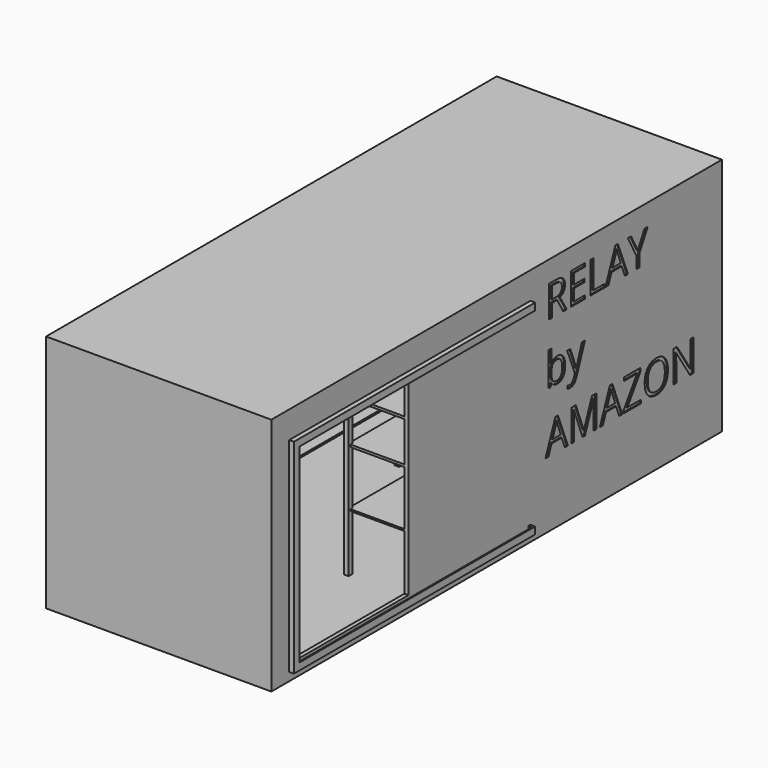
from build123d import *

# Parameters (mm, degrees)
F0_W          = 2438.4
F0_H          = 2590.8
F0_W_2        = 2352.04
F0_H_2        = 2395.22
F1_DEPTH      = 6096
F2_W          = 2352.04
F2_H          = 2395.22
F3_DEPTH      = 127
F4_W          = 2352.04
F4_H          = 2395.22
F5_DEPTH      = 127
F6_W          = 1524
F6_H          = 2032
F7_DEPTH      = 50.8
F9_DEPTH      = 50.8
F11_DEPTH     = 38.1
F12_TEXT_SIZE = 479.4042835551
F13_DEPTH     = 12.7
F14_W         = 50.8
F14_H         = 50.8
F15_DEPTH     = 2413
F18_DEPTH     = 19.05
F23_DEPTH     = 25.4
F24_DEPTH     = 25.4
F25_W         = 330.2
F25_H         = 228.6
F26_DEPTH     = 25.4
F27_W         = 353.0600027561
F27_H         = 251.4600027561
F27_W_2       = 330.2
F27_H_2       = 228.6
F28_DEPTH     = 2.54


# Not quite as in the source:
# - Text() gives the source's letters only with a copy of the font that has no kerning and outlines rounded to 1/6400 em; it was checked with that copy


with BuildPart() as f1:
    # F0 (on Front) → F1 (new body)
    with BuildSketch(Plane.XZ):
        Rectangle(F0_W, F0_H)
        with Locations((0, 54.61)):
            Rectangle(F0_W_2, F0_H_2, mode=Mode.SUBTRACT)
    extrude(amount=F1_DEPTH)

    # F2 (on face) → F3 (join)
    with BuildSketch(Plane(origin=(0, 0, 0), x_dir=(-1, 0, 0), z_dir=(0, 1, 0))):
        with Locations((0, 54.61)):
            Rectangle(F2_W, F2_H)
    extrude(amount=-F3_DEPTH)

    # F4 (on face) → F5 (join)
    with BuildSketch(Plane.XZ.offset(6096)):
        with Locations((0, 54.61)):
            Rectangle(F4_W, F4_H)
    extrude(amount=-F5_DEPTH)

    # F6 (on face) → F7 (cut)
    with BuildSketch(Plane.YZ.offset(1219.2)):
        with Locations((-5003.8, -114.3)):
            Rectangle(F6_W, F6_H)
    extrude(amount=-F7_DEPTH, mode=Mode.SUBTRACT)

    # F8 (on face) → F9 (join)
    with BuildSketch(Plane.YZ.offset(1219.2)):
        Polygon((-5765.8, -1130.3), (-5778.5, -1130.3), (-5778.5, 927.1), (-2590.8, 927.1), (-2590.8, 1003.3), (-5854.7, 1003.3), (-5854.7, -1206.5), (-2590.8, -1206.5), (-2590.8, -1130.3), (-4241.8, -1130.3), align=None)
    extrude(amount=F9_DEPTH)

    # F10 (on face) → F11 (cut)
    with BuildSketch(Plane.YZ.offset(1219.2)):
        Polygon((-2616.2, -1130.3), (-5778.5, -1130.3), (-5778.5, 927.1), (-2616.2, 927.1), (-2616.2, 977.9), (-5829.3, 977.9), (-5829.3, -1181.1), (-2616.2, -1181.1), align=None)
    extrude(amount=F11_DEPTH, mode=Mode.SUBTRACT)

    # F12 (on face) → F13 (cut)
    with BuildSketch(Plane.YZ.offset(1219.2)):
        with Locations((-2387.6, 721.6289158403)):
            Text('RELAY', F12_TEXT_SIZE, font='Open Sans', text_align=(TextAlign.LEFT, TextAlign.BOTTOM))
        with Locations((-2387.6, 69.6390902053)):
            Text('by', F12_TEXT_SIZE, font='Open Sans', text_align=(TextAlign.LEFT, TextAlign.BOTTOM))
        with Locations((-2387.6, -582.3507354296)):
            Text('AMAZON', F12_TEXT_SIZE, font='Open Sans', text_align=(TextAlign.LEFT, TextAlign.BOTTOM))
    extrude(amount=-F13_DEPTH, mode=Mode.SUBTRACT)


with BuildPart() as f15:
    # F14 (on face) → F15 (new body)
    with BuildSketch(Plane.XY.offset(-1143)):
        with Locations((-347.98, -889)):
            Rectangle(F14_W, F14_H)
    extrude(amount=F15_DEPTH)


with BuildPart() as f15b:
    # F14 (on face) → F15, piece 2 (new body)
    with BuildSketch(Plane.XY.offset(-1143)):
        with Locations((566.42, -889)):
            Rectangle(F14_W, F14_H)
    extrude(amount=F15_DEPTH)


with BuildPart() as f15c:
    # F14 (on face) → F15, piece 3 (new body)
    with BuildSketch(Plane.XY.offset(-1143)):
        with Locations((-347.98, -5664.2)):
            Rectangle(F14_W, F14_H)
    extrude(amount=F15_DEPTH)


with BuildPart() as f15d:
    # F14 (on face) → F15, piece 4 (new body)
    with BuildSketch(Plane.XY.offset(-1143)):
        with Locations((-347.98, -2413)):
            Rectangle(F14_W, F14_H)
    extrude(amount=F15_DEPTH)


with BuildPart() as f15e:
    # F14 (on face) → F15, piece 5 (new body)
    with BuildSketch(Plane.XY.offset(-1143)):
        with Locations((-347.98, -4140.2)):
            Rectangle(F14_W, F14_H)
    extrude(amount=F15_DEPTH)


with BuildPart() as f15f:
    # F14 (on face) → F15, piece 6 (new body)
    with BuildSketch(Plane.XY.offset(-1143)):
        with Locations((566.42, -2565.4)):
            Rectangle(F14_W, F14_H)
    extrude(amount=F15_DEPTH)


with BuildPart() as f15g:
    # F14 (on face) → F15, piece 7 (new body)
    with BuildSketch(Plane.XY.offset(-1143)):
        with Locations((566.42, -4241.8)):
            Rectangle(F14_W, F14_H)
    extrude(amount=F15_DEPTH)


with BuildPart() as f18:
    # F17 (on offset) → F18 (new body)
    with BuildSketch(Plane.XY.offset(-533.4)):
        Polygon((566.42, -889), (566.42, -4241.8), (1176.02, -4241.8), (1176.02, -127), (-1176.02, -127), (-1176.02, -5969), (515.62, -5969), (515.62, -5664.2), (-347.98, -5664.2), (-347.98, -889), align=None)
    extrude(amount=F18_DEPTH)


with BuildPart() as f23:
    # F20 (on offset) → F23 (new body)
    with BuildSketch(Plane.XY.offset(76.2)):
        Polygon((566.42, -889), (566.42, -4241.8), (1176.02, -4241.8), (1176.02, -127), (-1176.02, -127), (-1176.02, -5969), (515.62, -5969), (515.62, -5664.2), (-347.98, -5664.2), (-347.98, -889), align=None)
    extrude(amount=F23_DEPTH)


with BuildPart() as f24:
    # F22 (on offset) → F24 (new body)
    with BuildSketch(Plane.XY.offset(533.4)):
        Polygon((566.42, -889), (566.42, -4241.8), (1176.02, -4241.8), (1176.02, -127), (-1176.02, -127), (-1176.02, -5969), (515.62, -5969), (515.62, -5664.2), (-347.98, -5664.2), (-347.98, -889), align=None)
    extrude(amount=F24_DEPTH)


with BuildPart() as f26:
    # F25 (on face) → F26 (new body)
    with BuildSketch(Plane(origin=(0, -5969, 0), x_dir=(-1, 0, 0), z_dir=(0, 1, 0))):
        with Locations((-820.42, 76.2)):
            Rectangle(F25_W, F25_H)
    extrude(amount=F26_DEPTH)


with BuildPart() as f28:
    # F27 (on face) → F28 (new body)
    with BuildSketch(Plane(origin=(0, -5943.6, 0), x_dir=(-1, 0, 0), z_dir=(0, 1, 0))):
        with Locations((-820.42, 76.2)):
            Rectangle(F27_W, F27_H)
        with Locations((-820.42, 76.2)):
            Rectangle(F27_W_2, F27_H_2, mode=Mode.SUBTRACT)
    extrude(amount=-F28_DEPTH)


solid = Compound([f1.part, f15.part, f15b.part, f15c.part, f15d.part, f15e.part, f15f.part, f15g.part, f18.part, f23.part, f24.part, f26.part, f28.part])
